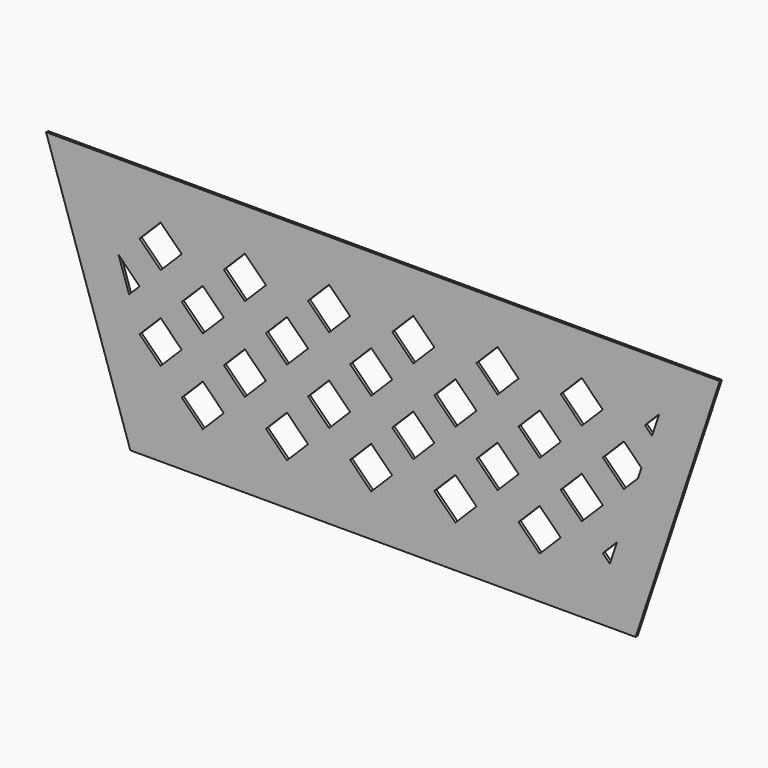
from build123d import *

# Parameters (mm, degrees)
F1_DEPTH = 3.175


# Not quite as in the source:
# - ends of sketch curves that miss each other by under 0.0002 mm in the source are joined


with BuildPart() as f1:
    # F0 (on Front) → F1 (new body)
    with BuildSketch(Plane.XZ):
        Polygon((406.4, 304.8), (0, 304.8), (-406.4, 304.8), (-304.8, 0), (0, 0), (304.8, 0), align=None)
        Polygon((-318.985431, 203.199999), (-335.918765, 254), (-268.185432, 254), (-166.585432, 254), (-64.985432, 254), (36.614568, 254), (138.214568, 254), (239.814568, 254), (335.918765, 254), (333.170855, 245.756271), (324.592716, 220.021853), (311.892716, 181.921853), (307.770855, 169.556269), (282.370863, 93.356295), (273.792716, 67.621853), (268.185432, 50.8), (189.014568, 50.8), (87.414568, 50.8), (-14.185432, 50.8), (-115.785432, 50.8), (-217.385432, 50.8), (-268.185432, 50.8), (-293.585431, 126.999998), (-306.285431, 165.099998), align=None, mode=Mode.SUBTRACT)
        Polygon((-268.185432, 254), (-335.918765, 254), (-318.985431, 203.199999), (-293.58543, 177.799999), (-306.285431, 165.099998), (-293.585431, 126.999998), (-268.185432, 50.8), (-217.385432, 50.8), (-115.785432, 50.8), (-14.185432, 50.8), (87.414568, 50.8), (189.014568, 50.8), (268.185432, 50.8), (273.792716, 67.621853), (265.214568, 76.2), (282.370863, 93.356295), (307.770855, 169.556269), (290.614577, 152.399991), (265.214576, 177.799992), (290.614576, 203.199992), (311.892716, 181.921853), (324.592716, 220.021853), (316.014576, 228.599992), (333.170855, 245.756271), (335.918765, 254), (239.814568, 254), (138.214568, 254), (36.614568, 254), (-64.985432, 254), (-166.585432, 254), align=None)
        Polygon((-191.985428, 76.199996), (-217.385432, 50.799993), (-242.785429, 76.199997), (-217.385429, 101.599997), align=None, mode=Mode.SUBTRACT)
        Polygon((-90.385427, 76.199995), (-115.785432, 50.79999), (-141.185427, 76.199996), (-115.785427, 101.599996), align=None, mode=Mode.SUBTRACT)
        Polygon((11.214575, 76.199994), (-14.185432, 50.799988), (-39.585426, 76.199994), (-14.185426, 101.599994), align=None, mode=Mode.SUBTRACT)
        Polygon((-268.185429, 101.599998), (-293.58543, 126.999998), (-268.18543, 152.399998), (-242.785429, 126.999998), align=None, mode=Mode.SUBTRACT)
        Polygon((-141.185428, 126.999996), (-166.585428, 101.599996), (-191.985429, 126.999997), (-166.585429, 152.399997), align=None, mode=Mode.SUBTRACT)
        Polygon((-39.585427, 126.999995), (-64.985427, 101.599995), (-90.385427, 126.999996), (-64.985427, 152.399996), align=None, mode=Mode.SUBTRACT)
        Polygon((112.814576, 76.199993), (87.414568, 50.799985), (62.014575, 76.199993), (87.414575, 101.599993), align=None, mode=Mode.SUBTRACT)
        Polygon((214.414577, 76.199991), (189.014568, 50.799983), (163.614576, 76.199992), (189.014576, 101.599992), align=None, mode=Mode.SUBTRACT)
        Polygon((62.014575, 126.999994), (36.614575, 101.599994), (11.214574, 126.999994), (36.614574, 152.399994), align=None, mode=Mode.SUBTRACT)
        Polygon((163.614576, 126.999993), (138.214576, 101.599993), (112.814575, 126.999993), (138.214575, 152.399993), align=None, mode=Mode.SUBTRACT)
        Polygon((239.814576, 152.399992), (265.214577, 126.999991), (239.814577, 101.599991), (214.414576, 126.999992), align=None, mode=Mode.SUBTRACT)
        Polygon((-242.78543, 177.799998), (-217.38543, 203.199998), (-191.985429, 177.799998), (-217.385429, 152.399998), align=None, mode=Mode.SUBTRACT)
        Polygon((-293.585431, 228.599999), (-268.185432, 254), (-242.78543, 228.599999), (-268.18543, 203.199999), align=None, mode=Mode.SUBTRACT)
        Polygon((-141.185429, 177.799997), (-115.785429, 203.199997), (-90.385428, 177.799996), (-115.785428, 152.399996), align=None, mode=Mode.SUBTRACT)
        Polygon((-39.585427, 177.799996), (-14.185427, 203.199996), (11.214573, 177.799995), (-14.185427, 152.399995), align=None, mode=Mode.SUBTRACT)
        Polygon((-191.98543, 228.599998), (-166.585432, 253.999996), (-141.185429, 228.599998), (-166.585429, 203.199998), align=None, mode=Mode.SUBTRACT)
        Polygon((-90.385429, 228.599997), (-64.985432, 253.999994), (-39.585428, 228.599996), (-64.985428, 203.199996), align=None, mode=Mode.SUBTRACT)
        Polygon((87.414574, 203.199994), (112.814575, 177.799994), (87.414575, 152.399994), (62.014574, 177.799994), align=None, mode=Mode.SUBTRACT)
        Polygon((163.614575, 177.799993), (189.014575, 203.199993), (214.414576, 177.799993), (189.014576, 152.399993), align=None, mode=Mode.SUBTRACT)
        Polygon((11.214573, 228.599996), (36.614568, 253.999991), (62.014573, 228.599995), (36.614573, 203.199995), align=None, mode=Mode.SUBTRACT)
        Polygon((112.814574, 228.599994), (138.214568, 253.999989), (163.614575, 228.599994), (138.214575, 203.199994), align=None, mode=Mode.SUBTRACT)
        Polygon((214.414575, 228.599993), (239.814568, 253.999986), (265.214576, 228.599993), (239.814576, 203.199993), align=None, mode=Mode.SUBTRACT)
    extrude(amount=F1_DEPTH)


solid = f1.part
